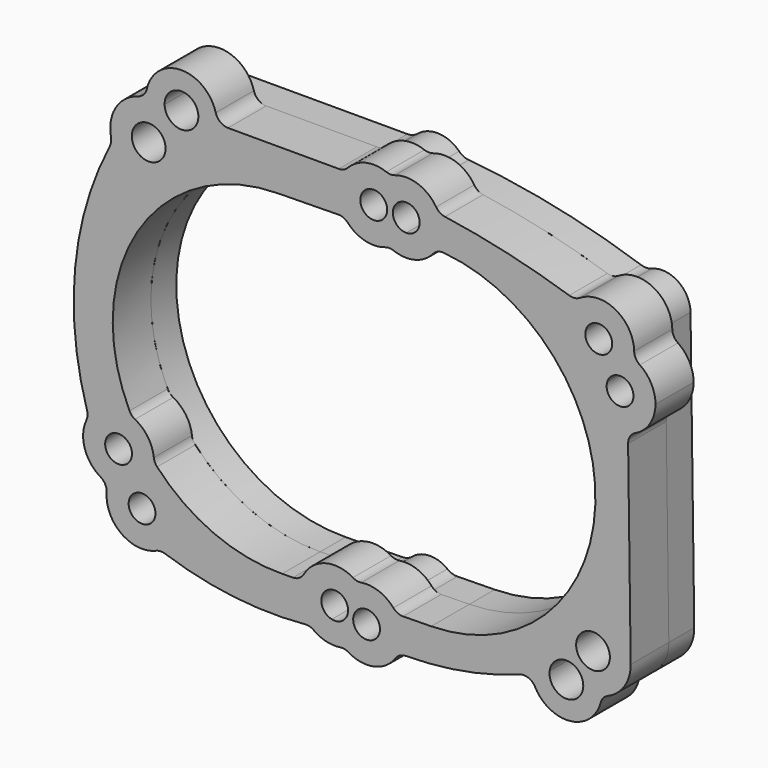
from build123d import *
from build123d import SkipClean  # not in build123d's __all__

# Parameters (mm, degrees)
F2_R     = 5.35813
F2_R_2   = 6.74624
F3_DEPTH = 12.7
F4_DEPTH = 19.05
F6_DEPTH = 19.05
F5_R     = 5.35813
F7_DEPTH = 25.4
F8_R     = 5.08


# Not quite as in the source:
# - a feature names something its author has since deleted; it is built from what else it names


with BuildPart() as f3:
    # F2 (on Front) → F3 (new body)
    with BuildSketch(Plane.XZ):
        with BuildLine():
            Line((43.9739345229, 72.9674244098), (-34.060832113, 72.9674244098))
            ThreePointArc((-34.060832113, 72.9674244098), (-45.8689494649, 67.4342536783), (-49.1731647113, 54.8195885878))
            ThreePointArc((-49.1731647113, 54.8195885878), (-49.1363008064, 52.7429754207), (-49.7714773161, 50.7655447658))
            ThreePointArc((-49.7714773161, 50.7655447658), (-64.019452698, -9.5986669756), (-48.3873339521, -69.6193277948))
            ThreePointArc((-48.3873339521, -69.6193277948), (-47.8355124841, -70.997156288), (-47.6186058759, -72.4654443431))
            ThreePointArc((-47.6186058759, -72.4654443431), (-43.7984217578, -80.4400964993), (-35.3242859421, -82.9655481192))
            ThreePointArc((-35.3242859421, -82.9655481192), (-33.768899146, -82.9580981146), (-32.2583615646, -83.3289886691))
            ThreePointArc((-32.2583615646, -83.3289886691), (3.3116441756, -91.6205047699), (39.8059532183, -90.1576462316))
            ThreePointArc((39.8059532183, -90.1576462316), (42.7500553961, -90.3338300006), (45.2969974228, -91.8210638983))
            ThreePointArc((45.2969974228, -91.8210638983), (53.2123481237, -94.9271772313), (61.0310405642, -91.5852069628))
            ThreePointArc((61.0310405642, -91.5852069628), (63.1537907079, -90.1629977205), (65.6652630564, -89.6926213347))
            ThreePointArc((65.6652630564, -89.6926213347), (97.7858423851, -86.3409596393), (128.1584963388, -75.3652070751))
            ThreePointArc((128.1584963388, -75.3652070751), (131.5205041438, -74.7013751888), (134.7378888972, -75.8812923901))
            ThreePointArc((134.7378888972, -75.8812923901), (150.5010785661, -77.0259521048), (158.610740004, -63.4604891285))
            Line((158.610740004, -63.4604891285), (157.1270137405, 47.0642682822))
            ThreePointArc((157.1270137405, 47.0642682822), (152.1224870362, 56.2966399376), (141.6815359098, 57.4229229811))
            ThreePointArc((141.6815359098, 57.4229229811), (139.5198972606, 56.9819236921), (137.3378340176, 57.307134434))
            ThreePointArc((137.3378340176, 57.307134434), (103.336647417, 66.544874537), (68.5025450606, 71.8365515379))
            ThreePointArc((68.5025450606, 71.8365515379), (66.4082980128, 72.4053728354), (64.627885221, 73.646162365))
            ThreePointArc((64.627885221, 73.646162365), (56.4648874082, 77.2254272018), (48.0070903171, 74.4127170444))
            ThreePointArc((48.0070903171, 74.4127170444), (46.1160839376, 73.3396576123), (43.9739345229, 72.9674244098))
        make_face()
        with Locations((-36.7124304175, -72.143279016)):
            Circle(F2_R, mode=Mode.SUBTRACT)
        with Locations((53.0443042517, -83.7169513106)):
            Circle(F2_R, mode=Mode.SUBTRACT)
        with Locations((143.548309803, -63.6626929045)):
            Circle(F2_R_2, mode=Mode.SUBTRACT)
        with BuildLine():
            ThreePointArc((43.6755138785, 56.846058352), (45.9105765729, 56.4757924543), (47.8734071208, 55.3444665406))
            ThreePointArc((47.8734071208, 55.3444665406), (56.0812953092, 52.40849438), (64.1963023198, 55.5922064049))
            ThreePointArc((64.1963023198, 55.5922064049), (66.1238954133, 56.7825790142), (68.3466918366, 57.2205038291))
            Line((68.3466918366, 57.2205038291), (76.8337704469, 57.3493160084))
            ThreePointArc((76.8337704469, 57.3493160084), (144.5129320112, -8.306166169), (78.8574498338, -75.9853277334))
            Line((78.8574498338, -75.9853277334), (63.9324369208, -76.2118513144))
            ThreePointArc((63.9324369208, -76.2118513144), (61.8187153718, -75.8836103275), (59.9339115407, -74.8721384049))
            ThreePointArc((59.9339115407, -74.8721384049), (52.8741621308, -72.5067570396), (45.8894488284, -75.0852974826))
            ThreePointArc((45.8894488284, -75.0852974826), (44.0362091952, -76.1535033589), (41.9334226593, -76.5457401707))
            Line((41.9334226593, -76.5457401707), (19.2511212272, -76.8899995812))
            ThreePointArc((19.2511212272, -76.8899995812), (-48.4280403371, -11.2345174038), (17.2274418403, 56.4446441606))
            Line((17.2274418403, 56.4446441606), (43.6755138785, 56.846058352))
        make_face(mode=Mode.SUBTRACT)
        with Locations((-34.060832113, 57.6012246311)):
            Circle(F2_R_2, mode=Mode.SUBTRACT)
        with Locations((55.8928772807, 64.8228377104)):
            Circle(F2_R, mode=Mode.SUBTRACT)
        with Locations((145.8289921284, 46.912599355)):
            Circle(F2_R, mode=Mode.SUBTRACT)
    extrude(amount=-F3_DEPTH)


with BuildPart() as f4:
    # F2 (on Front) → F4 (new body)
    with BuildSketch(Plane.XZ):
        with BuildLine():
            Line((43.9739345229, 72.9674244098), (-34.060832113, 72.9674244098))
            ThreePointArc((-34.060832113, 72.9674244098), (-45.8689494649, 67.4342536783), (-49.1731647113, 54.8195885878))
            ThreePointArc((-49.1731647113, 54.8195885878), (-49.1363008064, 52.7429754207), (-49.7714773161, 50.7655447658))
            ThreePointArc((-49.7714773161, 50.7655447658), (-64.019452698, -9.5986669756), (-48.3873339521, -69.6193277948))
            ThreePointArc((-48.3873339521, -69.6193277948), (-47.8355124841, -70.997156288), (-47.6186058759, -72.4654443431))
            ThreePointArc((-47.6186058759, -72.4654443431), (-43.7984217578, -80.4400964993), (-35.3242859421, -82.9655481192))
            ThreePointArc((-35.3242859421, -82.9655481192), (-33.768899146, -82.9580981146), (-32.2583615646, -83.3289886691))
            ThreePointArc((-32.2583615646, -83.3289886691), (3.3116441756, -91.6205047699), (39.8059532183, -90.1576462316))
            ThreePointArc((39.8059532183, -90.1576462316), (42.7500553961, -90.3338300006), (45.2969974228, -91.8210638983))
            ThreePointArc((45.2969974228, -91.8210638983), (53.2123481237, -94.9271772313), (61.0310405642, -91.5852069628))
            ThreePointArc((61.0310405642, -91.5852069628), (63.1537907079, -90.1629977205), (65.6652630564, -89.6926213347))
            ThreePointArc((65.6652630564, -89.6926213347), (97.7858423851, -86.3409596393), (128.1584963388, -75.3652070751))
            ThreePointArc((128.1584963388, -75.3652070751), (131.5205041438, -74.7013751888), (134.7378888972, -75.8812923901))
            ThreePointArc((134.7378888972, -75.8812923901), (150.5010785661, -77.0259521048), (158.610740004, -63.4604891285))
            Line((158.610740004, -63.4604891285), (157.1270137405, 47.0642682822))
            ThreePointArc((157.1270137405, 47.0642682822), (152.1224870362, 56.2966399376), (141.6815359098, 57.4229229811))
            ThreePointArc((141.6815359098, 57.4229229811), (139.5198972606, 56.9819236921), (137.3378340176, 57.307134434))
            ThreePointArc((137.3378340176, 57.307134434), (103.336647417, 66.544874537), (68.5025450606, 71.8365515379))
            ThreePointArc((68.5025450606, 71.8365515379), (66.4082980128, 72.4053728354), (64.627885221, 73.646162365))
            ThreePointArc((64.627885221, 73.646162365), (56.4648874082, 77.2254272018), (48.0070903171, 74.4127170444))
            ThreePointArc((48.0070903171, 74.4127170444), (46.1160839376, 73.3396576123), (43.9739345229, 72.9674244098))
        make_face()
        with Locations((-36.7124304175, -72.143279016)):
            Circle(F2_R, mode=Mode.SUBTRACT)
        with Locations((53.0443042517, -83.7169513106)):
            Circle(F2_R, mode=Mode.SUBTRACT)
        with Locations((143.548309803, -63.6626929045)):
            Circle(F2_R_2, mode=Mode.SUBTRACT)
        with BuildLine():
            ThreePointArc((43.6755138785, 56.846058352), (45.9105765729, 56.4757924543), (47.8734071208, 55.3444665406))
            ThreePointArc((47.8734071208, 55.3444665406), (56.0812953092, 52.40849438), (64.1963023198, 55.5922064049))
            ThreePointArc((64.1963023198, 55.5922064049), (66.1238954133, 56.7825790142), (68.3466918366, 57.2205038291))
            Line((68.3466918366, 57.2205038291), (76.8337704469, 57.3493160084))
            ThreePointArc((76.8337704469, 57.3493160084), (144.5129320112, -8.306166169), (78.8574498338, -75.9853277334))
            Line((78.8574498338, -75.9853277334), (63.9324369208, -76.2118513144))
            ThreePointArc((63.9324369208, -76.2118513144), (61.8187153718, -75.8836103275), (59.9339115407, -74.8721384049))
            ThreePointArc((59.9339115407, -74.8721384049), (52.8741621308, -72.5067570396), (45.8894488284, -75.0852974826))
            ThreePointArc((45.8894488284, -75.0852974826), (44.0362091952, -76.1535033589), (41.9334226593, -76.5457401707))
            Line((41.9334226593, -76.5457401707), (19.2511212272, -76.8899995812))
            ThreePointArc((19.2511212272, -76.8899995812), (-48.4280403371, -11.2345174038), (17.2274418403, 56.4446441606))
            Line((17.2274418403, 56.4446441606), (43.6755138785, 56.846058352))
        make_face(mode=Mode.SUBTRACT)
        with Locations((-34.060832113, 57.6012246311)):
            Circle(F2_R_2, mode=Mode.SUBTRACT)
        with Locations((55.8928772807, 64.8228377104)):
            Circle(F2_R, mode=Mode.SUBTRACT)
        with Locations((145.8289921284, 46.912599355)):
            Circle(F2_R, mode=Mode.SUBTRACT)
    extrude(amount=F4_DEPTH)

    # F5 (on face) → F6 (join, through all)
    with BuildSketch(Plane.XZ.offset(19.05)):
        with BuildLine():
            ThreePointArc((-31.7804118787, 63.9503535235), (-29.7032323577, 62.7512807968), (-28.176830892, 60.9012676261))
            ThreePointArc((-28.176830892, 60.9012676261), (-13.9896745727, 60.748746106), (-6.7783939823, 72.9674244098))
            Line((-6.7783939823, 72.9674244098), (-14.2063063776, 72.9674244098))
            ThreePointArc((-14.2063063776, 72.9674244098), (-20.9513446648, 66.3485132831), (-27.6963829519, 72.9674244098))
            Line((-27.6963829519, 72.9674244098), (-34.060832113, 72.9674244098))
            ThreePointArc((-34.060832113, 72.9674244098), (-34.5926931164, 72.9582171593), (-35.1239167497, 72.9306064417))
            ThreePointArc((-35.1239167497, 72.9306064417), (-34.2341052034, 68.1493497443), (-31.7804118787, 63.9503535235))
        make_face()
        with BuildLine():
            ThreePointArc((68.1880033695, 71.8739807488), (65.7833170775, 74.9750760997), (62.6204701677, 77.2979424248))
            ThreePointArc((62.6204701677, 77.2979424248), (61.6917486807, 76.7960656446), (60.8029573581, 76.2264571056))
            ThreePointArc((60.8029573581, 76.2264571056), (62.8363336959, 75.1155455508), (64.627885221, 73.646162365))
            ThreePointArc((64.627885221, 73.646162365), (66.2656326783, 72.474183155), (68.1880033695, 71.8739807488))
        make_face()
        with BuildLine():
            ThreePointArc((81.8658087677, 70.2882478503), (73.7404491625, 77.9040063562), (62.6204701677, 77.2979424248))
            ThreePointArc((62.6204701677, 77.2979424248), (65.7833170775, 74.9750760997), (68.1880033695, 71.8739807488))
            ThreePointArc((68.1880033695, 71.8739807488), (68.3450407908, 71.8533045294), (68.5025450606, 71.8365515379))
            ThreePointArc((68.5025450606, 71.8365515379), (75.1926362811, 71.1354116954), (81.8658087677, 70.2882478503))
        make_face()
        with BuildLine():
            ThreePointArc((67.8370340994, 57.1922504735), (65.3473355799, 54.2633887685), (62.1621928224, 52.1112514079))
            ThreePointArc((62.1621928224, 52.1112514079), (72.6340279689, 50.9163380685), (81.0353777762, 57.2806503359))
            ThreePointArc((81.0353777762, 57.2806503359), (78.9351151996, 57.3480919964), (76.8337704469, 57.3493160084))
            Line((76.8337704469, 57.3493160084), (68.3466918366, 57.2205038291))
            ThreePointArc((68.3466918366, 57.2205038291), (68.0915789625, 57.2115002807), (67.8370340994, 57.1922504735))
        make_face()
        with BuildLine():
            ThreePointArc((168.5230112633, 31.3309720818), (166.1369044227, 39.2015230625), (159.7819841572, 44.4220658517))
            ThreePointArc((159.7819841572, 44.4220658517), (158.8520682327, 41.3190108405), (157.2418743919, 38.5081444573))
            Line((157.2418743919, 38.5081444573), (157.2779878668, 35.8180033217))
            ThreePointArc((157.2779878668, 35.8180033217), (159.0612206249, 33.8822734663), (159.7076186352, 31.3309720818))
            ThreePointArc((159.7076186352, 31.3309720818), (159.095042674, 28.8431469349), (157.3973820559, 26.9241702037))
            Line((157.3973820559, 26.9241702037), (157.5236614252, 17.5174507788))
            ThreePointArc((157.5236614252, 17.5174507788), (165.4372736609, 22.5020555621), (168.5230112633, 31.3309720818))
        make_face()
        with BuildLine():
            ThreePointArc((118.9380409893, -79.5952083516), (133.5455993884, -91.3273110011), (147.0290133148, -78.3188313109))
            ThreePointArc((147.0290133148, -78.3188313109), (143.2917294447, -78.7242949589), (139.5704245601, -78.1917712965))
            ThreePointArc((139.5704245601, -78.1917712965), (131.9720438311, -83.8501971726), (126.2081251094, -76.3315261419))
            ThreePointArc((126.2081251094, -76.3315261419), (122.5974703303, -78.0176916486), (118.9380409893, -79.5952083516))
        make_face()
        with BuildLine():
            ThreePointArc((40.3809353006, -90.0830985361), (42.0481146912, -92.6596890815), (44.2308305712, -94.8170155164))
            ThreePointArc((44.2308305712, -94.8170155164), (45.8840655988, -94.2253558535), (47.4514553846, -93.4338152844))
            ThreePointArc((47.4514553846, -93.4338152844), (46.3256600241, -92.6923189175), (45.2969974228, -91.8210638983))
            ThreePointArc((45.2969974228, -91.8210638983), (43.0255821621, -90.4242140411), (40.3809353006, -90.0830985361))
        make_face()
        with BuildLine():
            ThreePointArc((39.8059532183, -90.1576462316), (35.1733959424, -90.892774504), (30.5182650816, -91.4678894144))
            ThreePointArc((30.5182650816, -91.4678894144), (36.9279640515, -94.970932216), (44.2308305712, -94.8170155164))
            ThreePointArc((44.2308305712, -94.8170155164), (42.0481146912, -92.6596890815), (40.3809353006, -90.0830985361))
            ThreePointArc((40.3809353006, -90.0830985361), (40.092592982, -90.1138065299), (39.8059532183, -90.1576462316))
        make_face()
        with BuildLine():
            ThreePointArc((49.1042989114, -70.1020660152), (36.223906761, -67.6246150637), (26.8264467697, -76.775025485))
            Line((26.8264467697, -76.775025485), (37.5256625239, -76.6126387131))
            ThreePointArc((37.5256625239, -76.6126387131), (39.3037271725, -75.935708806), (41.2062467615, -75.9227779389))
            ThreePointArc((41.2062467615, -75.9227779389), (44.6355594883, -72.3072293511), (49.1042989114, -70.1020660152))
        make_face()
        with BuildLine():
            ThreePointArc((-31.9191932881, -54.1508352923), (-34.3932648991, -46.217236235), (-40.8894056468, -41.0342660708))
            ThreePointArc((-40.8894056468, -41.0342660708), (-36.7964526911, -47.8607380127), (-31.9191932881, -54.1508352923))
        make_face()
        with BuildLine():
            ThreePointArc((-49.8558138695, -66.8385438555), (-54.4089622052, -56.9454834698), (-58.1096425641, -46.7029853154))
            ThreePointArc((-58.1096425641, -46.7029853154), (-59.3625108122, -59.1978571529), (-50.1988715034, -67.7838466532))
            ThreePointArc((-50.1988715034, -67.7838466532), (-50.0357291109, -67.3081517566), (-49.8558138695, -66.8385438555))
        make_face()
        with BuildLine():
            Line((-14.2063063776, 72.9674244098), (-6.7783939823, 72.9674244098))
            ThreePointArc((-6.7783939823, 72.9674244098), (-6.7779650238, 73.0310882042), (-6.7778220367, 73.0947532831))
            ThreePointArc((-6.7778220367, 73.0947532831), (-21.0334194616, 87.2680382734), (-35.1239167497, 72.9306064417))
            ThreePointArc((-35.1239167497, 72.9306064417), (-34.5926931164, 72.9582171593), (-34.060832113, 72.9674244098))
            Line((-34.060832113, 72.9674244098), (-27.6963829519, 72.9674244098))
            ThreePointArc((-27.6963829519, 72.9674244098), (-21.0150119367, 79.8406928482), (-14.2051046648, 73.0947532831))
            ThreePointArc((-14.2051046648, 73.0947532831), (-14.2054050997, 73.0310860111), (-14.2063063776, 72.9674244098))
        make_face()
        with BuildLine():
            ThreePointArc((62.6204701677, 77.2979424248), (52.6385562551, 78.617696838), (44.2989654589, 72.9757483781))
            ThreePointArc((44.2989654589, 72.9757483781), (46.2684208774, 73.3964589168), (48.0070903171, 74.4127170444))
            ThreePointArc((48.0070903171, 74.4127170444), (54.1504304033, 77.1157340557), (60.8029573581, 76.2264571056))
            ThreePointArc((60.8029573581, 76.2264571056), (61.6917486807, 76.7960656446), (62.6204701677, 77.2979424248))
        make_face()
        with BuildLine():
            ThreePointArc((47.8734071208, 55.3444665406), (46.1491573991, 56.3850024121), (44.1857942955, 56.8332850529))
            ThreePointArc((44.1857942955, 56.8332850529), (52.2919428008, 51.114372641), (62.1621928224, 52.1112514079))
            ThreePointArc((62.1621928224, 52.1112514079), (61.2523435389, 52.6465813848), (60.3848619621, 53.2481456929))
            ThreePointArc((60.3848619621, 53.2481456929), (53.8411880439, 52.5777573532), (47.8734071208, 55.3444665406))
        make_face()
        with BuildLine():
            ThreePointArc((60.3848619621, 53.2481456929), (61.2523435389, 52.6465813848), (62.1621928224, 52.1112514079))
            ThreePointArc((62.1621928224, 52.1112514079), (65.3473355799, 54.2633887685), (67.8370340994, 57.1922504735))
            ThreePointArc((67.8370340994, 57.1922504735), (65.8881797655, 56.6845903629), (64.1963023198, 55.5922064049))
            ThreePointArc((64.1963023198, 55.5922064049), (62.3970515276, 54.2470569334), (60.3848619621, 53.2481456929))
        make_face()
        with BuildLine():
            ThreePointArc((160.0025147564, 46.912599355), (151.6897331974, 59.8176548686), (136.5022936497, 57.5850610755))
            ThreePointArc((136.5022936497, 57.5850610755), (136.9201632155, 57.4463965297), (137.3378340176, 57.307134434))
            ThreePointArc((137.3378340176, 57.307134434), (139.5198972606, 56.9819236921), (141.6815359098, 57.4229229811))
            ThreePointArc((141.6815359098, 57.4229229811), (152.1224870362, 56.2966399376), (157.1270137405, 47.0642682822))
            Line((157.1270137405, 47.0642682822), (157.1517084975, 45.2247227465))
            ThreePointArc((157.1517084975, 45.2247227465), (158.4863592988, 44.8873375535), (159.7819841572, 44.4220658517))
            ThreePointArc((159.7819841572, 44.4220658517), (159.9472744591, 45.6624602751), (160.0025147564, 46.912599355))
        make_face()
        with BuildLine():
            ThreePointArc((157.2418743919, 38.5081444573), (158.8520682327, 41.3190108405), (159.7819841572, 44.4220658517))
            ThreePointArc((159.7819841572, 44.4220658517), (158.4863592988, 44.8873375535), (157.1517084975, 45.2247227465))
            Line((157.1517084975, 45.2247227465), (157.2418743919, 38.5081444573))
        make_face()
        with BuildLine():
            ThreePointArc((51.5587623657, -72.6043202433), (50.4091790564, -71.2770277253), (49.1042989114, -70.1020660152))
            ThreePointArc((49.1042989114, -70.1020660152), (44.6355594883, -72.3072293511), (41.2062467615, -75.9227779389))
            ThreePointArc((41.2062467615, -75.9227779389), (42.0287438691, -76.1336791851), (42.807596764, -76.4718640396))
            ThreePointArc((42.807596764, -76.4718640396), (44.4424556537, -75.9873606206), (45.8894488284, -75.0852974826))
            ThreePointArc((45.8894488284, -75.0852974826), (48.549537469, -73.4459009503), (51.5587623657, -72.6043202433))
        make_face()
        with BuildLine():
            Line((63.9324369208, -76.2118513144), (65.0570360047, -76.1947827723))
            ThreePointArc((65.0570360047, -76.1947827723), (58.101232895, -70.4762482936), (49.1042989114, -70.1020660152))
            ThreePointArc((49.1042989114, -70.1020660152), (50.4091790564, -71.2770277253), (51.5587623657, -72.6043202433))
            ThreePointArc((51.5587623657, -72.6043202433), (55.9746166111, -72.8951828133), (59.9339115407, -74.8721384049))
            ThreePointArc((59.9339115407, -74.8721384049), (61.8187153718, -75.8836103275), (63.9324369208, -76.2118513144))
        make_face()
        with BuildLine():
            ThreePointArc((47.4514553846, -93.4338152844), (45.8840655988, -94.2253558535), (44.2308305712, -94.8170155164))
            ThreePointArc((44.2308305712, -94.8170155164), (56.3045885659, -97.5104022885), (65.894776882, -89.6964242695))
            ThreePointArc((65.894776882, -89.6964242695), (65.7800191508, -89.694572191), (65.6652630564, -89.6926213347))
            ThreePointArc((65.6652630564, -89.6926213347), (63.1537907079, -90.1629977205), (61.0310405642, -91.5852069628))
            ThreePointArc((61.0310405642, -91.5852069628), (54.5565914126, -94.8259742865), (47.4514553846, -93.4338152844))
        make_face()
        with BuildLine():
            ThreePointArc((-49.8558138695, -66.8385438555), (-50.0357291109, -67.3081517566), (-50.1988715034, -67.7838466532))
            ThreePointArc((-50.1988715034, -67.7838466532), (-49.7177945496, -67.9202524105), (-49.2322053452, -68.0396035339))
            ThreePointArc((-49.2322053452, -68.0396035339), (-49.5455878698, -67.4398931526), (-49.8558138695, -66.8385438555))
        make_face()
        with BuildLine():
            ThreePointArc((-49.2322053452, -68.0396035339), (-49.7177945496, -67.9202524105), (-50.1988715034, -67.7838466532))
            ThreePointArc((-50.1988715034, -67.7838466532), (-45.5670686099, -83.2105336969), (-29.5000091999, -84.3444971465))
            ThreePointArc((-29.5000091999, -84.3444971465), (-30.8819260107, -83.8441870788), (-32.2583615646, -83.3289886691))
            ThreePointArc((-32.2583615646, -83.3289886691), (-33.768899146, -82.9580981146), (-35.3242859421, -82.9655481192))
            ThreePointArc((-35.3242859421, -82.9655481192), (-43.7984217578, -80.4400964993), (-47.6186058759, -72.4654443431))
            ThreePointArc((-47.6186058759, -72.4654443431), (-47.8355124841, -70.997156288), (-48.3873339521, -69.6193277948))
            ThreePointArc((-48.3873339521, -69.6193277948), (-48.8125176086, -68.8309353339), (-49.2322053452, -68.0396035339))
        make_face()
    extrude(amount=-F6_DEPTH)

    # F5 (on face) → F7 (cut)
    with BuildSketch(Plane.XZ.offset(19.05)):
        with BuildLine():
            ThreePointArc((-27.6963829519, 72.9674244098), (-20.9513446648, 66.3485132831), (-14.2063063776, 72.9674244098))
            Line((-14.2063063776, 72.9674244098), (-27.6963829519, 72.9674244098))
        make_face()
        with BuildLine():
            ThreePointArc((70.0663999088, 64.8228377104), (69.8253606799, 67.4256534969), (69.1104413661, 69.9399407324))
            ThreePointArc((69.1104413661, 69.9399407324), (63.5325424365, 64.6838323339), (68.9155405049, 59.2282880201))
            ThreePointArc((68.9155405049, 59.2282880201), (69.7757040025, 61.9669900427), (70.0663999088, 64.8228377104))
        make_face()
        with BuildLine():
            ThreePointArc((74.2479157094, 64.5863561222), (72.7557822686, 68.2962924696), (69.1104413661, 69.9399407324))
            ThreePointArc((69.1104413661, 69.9399407324), (69.8253606799, 67.4256534969), (70.0663999088, 64.8228377104))
            ThreePointArc((70.0663999088, 64.8228377104), (69.7757040025, 61.9669900427), (68.9155405049, 59.2282880201))
            ThreePointArc((68.9155405049, 59.2282880201), (72.6876505464, 60.8067027284), (74.2479157094, 64.5863561222))
        make_face()
        with BuildLine():
            ThreePointArc((155.5112595377, 36.5616360422), (152.6291895279, 34.476922493), (149.3188300517, 33.1754317082))
            ThreePointArc((149.3188300517, 33.1754317082), (151.0704023262, 27.0933843158), (157.3973820559, 26.9241702037))
            Line((157.3973820559, 26.9241702037), (157.2779878668, 35.8180033217))
            ThreePointArc((157.2779878668, 35.8180033217), (156.4281480225, 36.2694670194), (155.5112595377, 36.5616360422))
        make_face()
        with BuildLine():
            ThreePointArc((155.5112595377, 36.5616360422), (151.7787556814, 36.0321303622), (149.3188300517, 33.1754317082))
            ThreePointArc((149.3188300517, 33.1754317082), (152.6291895279, 34.476922493), (155.5112595377, 36.5616360422))
        make_face()
        with BuildLine():
            Line((40.8088235755, -76.5628087128), (37.5256625239, -76.6126387131))
            ThreePointArc((37.5256625239, -76.6126387131), (35.003095551, -82.0678506895), (39.133608465, -86.4338036104))
            ThreePointArc((39.133608465, -86.4338036104), (39.0705871022, -81.3454596463), (40.8088235755, -76.5628087128))
        make_face()
        with BuildLine():
            ThreePointArc((40.8088235755, -76.5628087128), (39.0705871022, -81.3454596463), (39.133608465, -86.4338036104))
            ThreePointArc((39.133608465, -86.4338036104), (43.6456008737, -85.3800528487), (45.6489552309, -81.202130221))
            ThreePointArc((45.6489552309, -81.202130221), (44.8840129122, -78.443111551), (42.807596764, -76.4718640396))
            ThreePointArc((42.807596764, -76.4718640396), (42.3717870405, -76.5239166999), (41.9334226593, -76.5457401707))
            Line((41.9334226593, -76.5457401707), (40.8088235755, -76.5628087128))
        make_face()
        with BuildLine():
            ThreePointArc((134.7378888972, -75.8812923901), (137.0506354704, -77.2530541283), (139.5704245601, -78.1917712965))
            ThreePointArc((139.5704245601, -78.1917712965), (139.6289505757, -77.6815708579), (139.6484970032, -77.1683966973))
            ThreePointArc((139.6484970032, -77.1683966973), (133.3215026297, -70.4351963258), (126.2081251094, -76.3315261419))
            ThreePointArc((126.2081251094, -76.3315261419), (127.1852825317, -75.8523464086), (128.1584963388, -75.3652070751))
            ThreePointArc((128.1584963388, -75.3652070751), (131.5205041438, -74.7013751888), (134.7378888972, -75.8812923901))
        make_face()
        with Locations((-46.0925558535, -54.2181946058)):
            Circle(F5_R)
    with SkipClean():  # cleaning this boolean's faces spoils the solid; the shape is the same uncleaned
        extrude(amount=-F7_DEPTH, mode=Mode.SUBTRACT)

    # F8
    f8_edges = [f4.edges().sort_by_distance(p)[0] for p in [
        (136.502294, -9.525, 57.585061),
        (159.781984, -9.525, 44.422066),
        (157.523661, -9.525, 17.517451),
        (147.029013, -9.525, -78.318831),
        (118.938041, -9.525, -79.595208),
        (65.894777, -9.525, -89.696424),
        (49.104299, -9.525, -70.102066),
        (30.518265, -9.525, -91.467889),
        (65.057036, -9.525, -76.194783),
        (44.230831, -9.525, -94.817016),
        (26.826447, -9.525, -76.775025),
        (-29.500009, -9.525, -84.344497),
        (-50.198872, -9.525, -67.783847),
        (-58.109643, -9.525, -46.702985),
        (-31.919193, -9.525, -54.150835),
        (-40.889406, -9.525, -41.034266),
        (62.62047, -9.525, 77.297942),
        (81.865809, -9.525, 70.288248),
        (44.298965, -9.525, 72.975748),
        (44.185794, -9.525, 56.833285),
        (62.162193, -9.525, 52.111251),
        (81.035378, -9.525, 57.28065),
        (-6.778394, -9.525, 72.967424),
        (-35.123917, -9.525, 72.930606),
    ]]
    fillet(f8_edges, radius=F8_R)


solid = Compound([f3.part, f4.part])
